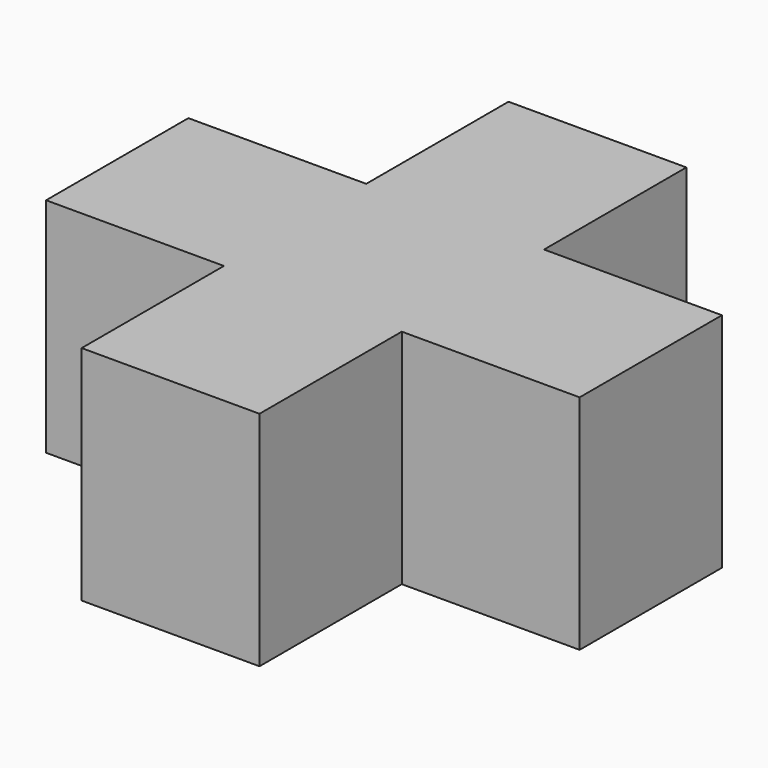
from build123d import *

# Parameters (mm, degrees)
F0_W     = 20
F0_H     = 20
F1_DEPTH = 25


with BuildPart() as f1:
    # F0 (on Top) → F1 (new body)
    with BuildSketch(Plane.XY):
        with Locations((10, 10)):
            Rectangle(F0_W, F0_H)
        Polygon((-20, 20), (0, 20), (0, 30), (0, 40), (-20, 40), align=None)
        Polygon((0, 30), (0, 20), (20, 20), (20, 40), (0, 40), align=None)
        with Locations((30, 30)):
            Rectangle(F0_W, F0_H)
        with Locations((10, 50)):
            Rectangle(F0_W, F0_H)
    extrude(amount=F1_DEPTH)


solid = f1.part
